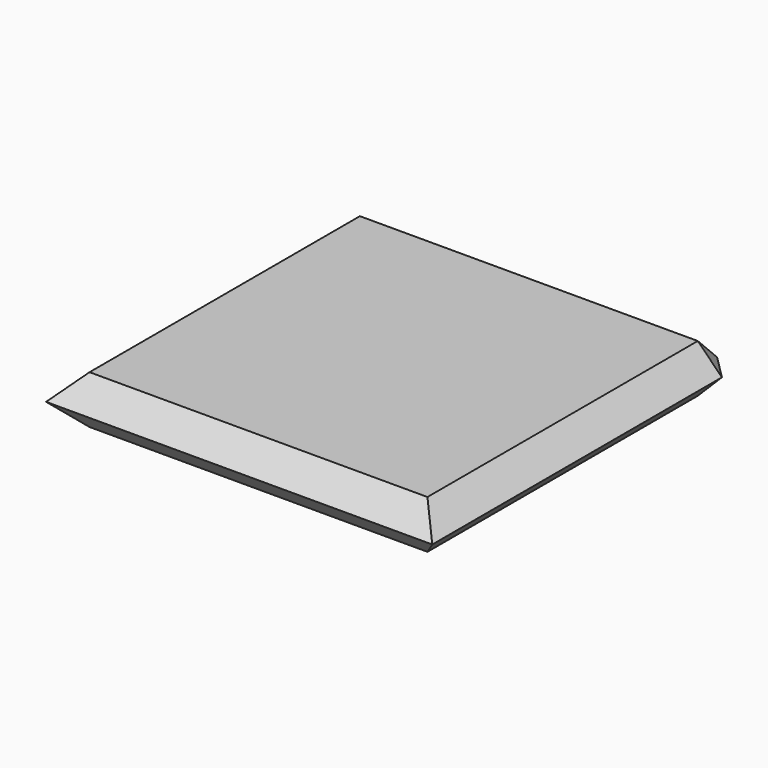
from build123d import *

# Parameters (mm, degrees)
F0_W     = 80
F0_H     = 80
F1_DEPTH = 10
F2_SIZE  = 4.99999


# Not quite as in the source:
# - a fillet or chamfer is up to 0.001 mm smaller than in the source, because OpenCascade refuses the exact size


with BuildPart() as f1:
    # F0 (on Top) → F1 (new body)
    with BuildSketch(Plane.XY):
        with Locations((40, -40)):
            Rectangle(F0_W, F0_H)
    extrude(amount=F1_DEPTH)

    # F2 (size 5 in the source; OpenCascade refuses exactly that, so slightly less here)
    f2_edges = [f1.edges().sort_by_distance(p)[0] for p in [
        (40, 0, 0),
        (40, 0, 10),
        (0, 0, 5),
        (80, 0, 5),
        (80, -40, 0),
        (80, -40, 10),
        (40, -80, 0),
        (40, -80, 10),
        (0, -40, 0),
        (0, -40, 10),
    ]]
    chamfer(f2_edges, length=F2_SIZE)


solid = f1.part
